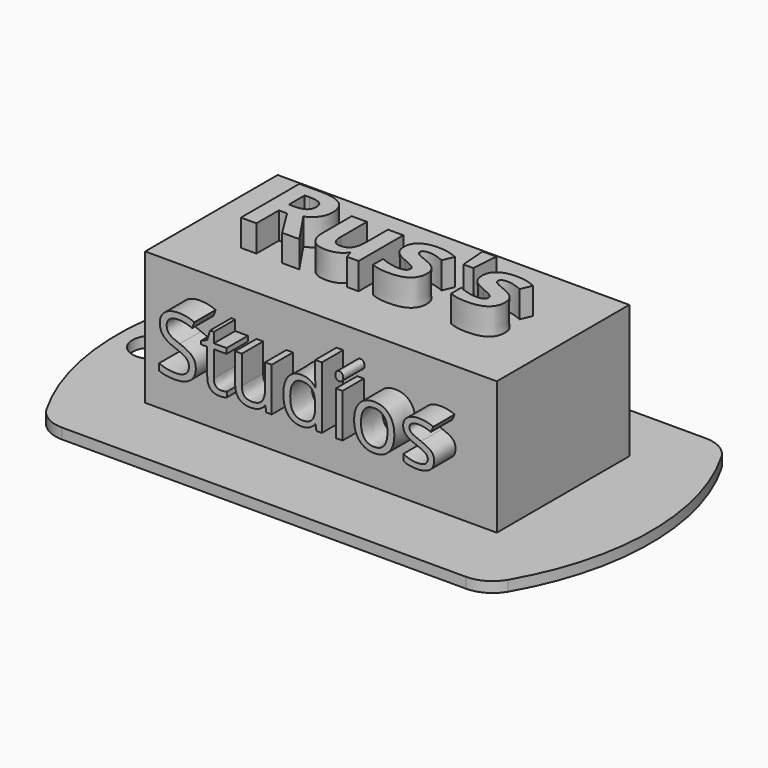
from build123d import *

# Parameters (mm, degrees)
F0_R         = 1.8739594118
F1_DEPTH     = 1
F2_W         = 33.5064027458
F2_H         = 15.779693611
F3_DEPTH     = 12.7
F4_TEXT_SIZE = 9.7528197744
F5_DEPTH     = 2.54
F6_TEXT_SIZE = 7.7908548216
F7_DEPTH     = 2.54


# Not quite as in the source:
# - Text() gives the source's letters only with a copy of the font that has no kerning and outlines rounded to 1/6400 em; it was checked with that copy


with BuildPart() as f1:
    # F0 (on Top) → F1 (new body)
    with BuildSketch(Plane.XY):
        with BuildLine():
            ThreePointArc((-19.2474145991, 14.2875), (-20.8349145991, 13.862130657), (-21.9970452561, 12.7))
            ThreePointArc((-21.9970452561, 12.7), (-25.4, 0), (-21.9970452561, -12.7))
            ThreePointArc((-21.9970452561, -12.7), (-20.8349145991, -13.862130657), (-19.2474145991, -14.2875))
            Line((-19.2474145991, -14.2875), (19.2474145991, -14.2875))
            ThreePointArc((19.2474145991, -14.2875), (20.8349145991, -13.862130657), (21.9970452561, -12.7))
            ThreePointArc((21.9970452561, -12.7), (25.4, 0), (21.9970452561, 12.7))
            ThreePointArc((21.9970452561, 12.7), (20.8349145991, 13.862130657), (19.2474145991, 14.2875))
            Line((19.2474145991, 14.2875), (-19.2474145991, 14.2875))
        make_face()
        with Locations((-22.0978986472, 0)):
            Circle(F0_R, mode=Mode.SUBTRACT)
    extrude(amount=F1_DEPTH)


with BuildPart() as f3:
    # F2 (on face) → F3 (new body)
    with BuildSketch(Plane.XY.offset(1)):
        with Locations((-0.1605348662, 0.5833026953)):
            Rectangle(F2_W, F2_H)
    extrude(amount=F3_DEPTH)

    # F4 (on face) → F5 (join)
    with BuildSketch(Plane.XY.offset(13.7)):
        with Locations((-12.5834839419, -2.4062009114)):
            Text("Rus's", F4_TEXT_SIZE, font='Open Sans', font_style=FontStyle.BOLD, text_align=(TextAlign.LEFT, TextAlign.BOTTOM))
    extrude(amount=F5_DEPTH)

    # F6 (on face) → F7 (join)
    with BuildSketch(Plane.XZ.offset(7.3065441102)):
        with Locations((-13.9592951164, 5.6398892775)):
            Text('Studios', F6_TEXT_SIZE, font='Open Sans', text_align=(TextAlign.LEFT, TextAlign.BOTTOM))
    extrude(amount=F7_DEPTH)


solid = Compound([f1.part, f3.part])
